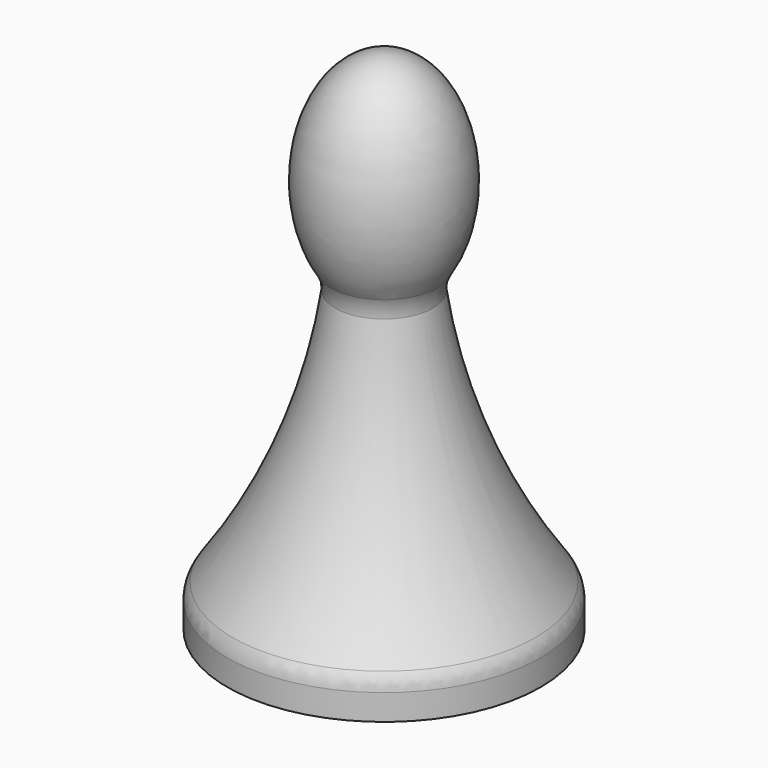
from build123d import *

# Parameters (mm, degrees)
F2_R = 2.54


with BuildPart() as f1:
    # F0 (on Front) → F1 (revolve)
    with BuildSketch(Plane.XZ):
        with BuildLine():
            ThreePointArc((-4.318, 28.2435778242), (-7.6873775939, 15.0668729236), (-14.2875, 3.175))
            Line((-14.2875, 3.175), (-14.2875, 0))
            Line((-14.2875, 0), (-7.3279, 0))
            Line((-7.3279, 0), (-7.3279, 9.906))
            Line((-7.3279, 9.906), (-3.556, 13.6779))
            Line((-3.556, 13.6779), (-3.556, 22.5698975516))
            ThreePointArc((-3.556, 22.5698975516), (-3.3626540126, 23.5419134698), (-2.8120512242, 24.3659487758))
            Line((-2.8120512242, 24.3659487758), (0, 27.178))
            Line((0, 27.178), (0, 46.228))
            add(Edge.make_bspline(
                [(0, 46.228), (-18.7837371747, 46.228), (-4.318, 28.2435778242)],
                knots=[0, 0, 0, 2.4498260338, 2.4498260338, 2.4498260338], degree=2, weights=[1, 0.3390278065, 1]))
        make_face()
    revolve(axis=Axis((0, 0, 36.703), (0, 0, -1)))

    # F2
    f2_edges = [f1.edges().sort_by_distance(p)[0] for p in [
        (4.318, 0, 28.243578),
        (14.2875, 0, 3.175),
    ]]
    fillet(f2_edges, radius=F2_R)


solid = f1.part
